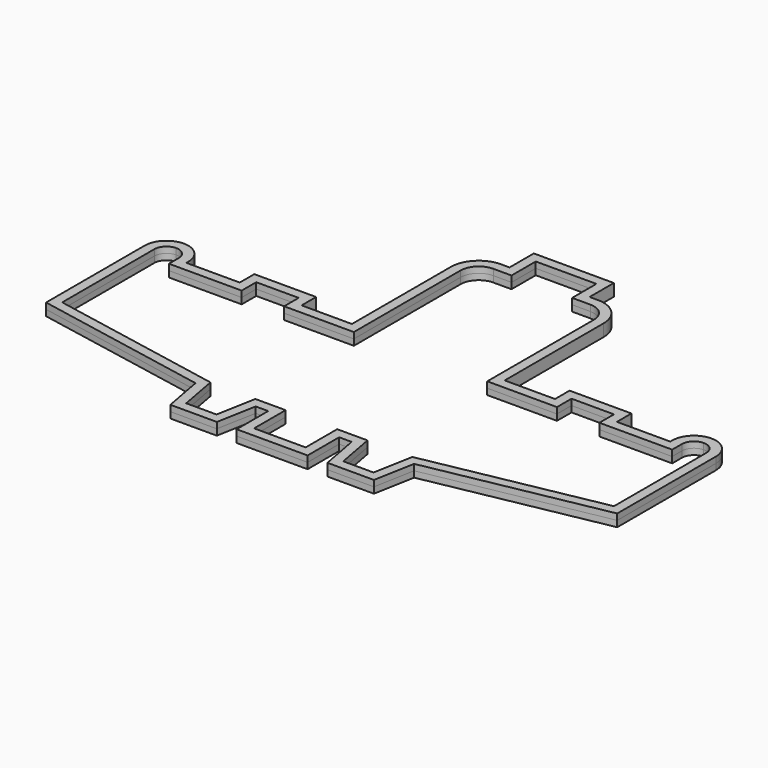
from build123d import *

# Parameters (mm, degrees)
F1_DEPTH = 1


# Not quite as in the source:
# - a feature names something its author has since deleted; it is built from what else it names


with BuildPart() as f1:
    # F0 (on Top) → F1 (new body, symmetric)
    with BuildSketch(Plane.XY):
        with BuildLine():
            Line((6.5999999642, 31.0999999642), (0, 31.0999999642))
            Line((0, 31.0999999642), (-6.5999999642, 31.0999999642))
            Line((-6.5999999642, 31.0999999642), (-6.5999999642, 26.0999999642))
            Line((-6.5999999642, 26.0999999642), (-8, 26.0999999642))
            ThreePointArc((-8, 26.0999999642), (-11.2526911682, 24.7526911682), (-12.5999999642, 21.5))
            Line((-12.5999999642, 21.5), (-12.5999999642, 1.0999999642))
            Line((-12.5999999642, 1.0999999642), (-20.9000000358, 1.0999999642))
            Line((-20.9000000358, 1.0999999642), (-20.9000000358, 4.0999999642))
            Line((-20.9000000358, 4.0999999642), (-31.0999999642, 4.0999999642))
            Line((-31.0999999642, 4.0999999642), (-31.0999999642, 1.0999999642))
            Line((-31.0999999642, 1.0999999642), (-39.922291276, 1.0999999642))
            ThreePointArc((-39.922291276, 1.0999999642), (-40.8167184403, 3.8999999613), (-43.5, 5.0999999642))
            ThreePointArc((-43.5, 5.0999999642), (-46.045584387, 4.045584387), (-47.0999999642, 1.5))
            Line((-47.0999999642, 1.5), (-47.0999999642, -18.823789758))
            Line((-47.0999999642, -18.823789758), (-18.0247169235, -24.366737998))
            Line((-18.0247169235, -24.366737998), (-16.7816531759, -31.0999999642))
            Line((-16.7816531759, -31.0999999642), (-9.1183468241, -31.0999999642))
            Line((-9.1183468241, -31.0999999642), (-7.9183468241, -24.5999999642))
            Line((-7.9183468241, -24.5999999642), (-5.8499999642, -24.5999999642))
            Line((-5.8499999642, -24.5999999642), (-5.8499999642, -31.0999999642))
            Line((-5.8499999642, -31.0999999642), (0, -31.0999999642))
            Line((0, -31.0999999642), (5.8499999642, -31.0999999642))
            Line((5.8499999642, -31.0999999642), (5.8499999642, -24.5999999642))
            Line((5.8499999642, -24.5999999642), (7.9183468241, -24.5999999642))
            Line((7.9183468241, -24.5999999642), (9.1183468241, -31.0999999642))
            Line((9.1183468241, -31.0999999642), (16.7816531759, -31.0999999642))
            Line((16.7816531759, -31.0999999642), (18.0247169235, -24.366737998))
            Line((18.0247169235, -24.366737998), (47.0999999642, -18.823789758))
            Line((47.0999999642, -18.823789758), (47.0999999642, 1.5))
            ThreePointArc((47.0999999642, 1.5), (46.045584387, 4.045584387), (43.5, 5.0999999642))
            ThreePointArc((43.5, 5.0999999642), (40.8167184403, 3.8999999613), (39.922291276, 1.0999999642))
            Line((39.922291276, 1.0999999642), (31.0999999642, 1.0999999642))
            Line((31.0999999642, 1.0999999642), (31.0999999642, 4.0999999642))
            Line((31.0999999642, 4.0999999642), (20.9000000358, 4.0999999642))
            Line((20.9000000358, 4.0999999642), (20.9000000358, 1.0999999642))
            Line((20.9000000358, 1.0999999642), (12.5999999642, 1.0999999642))
            Line((12.5999999642, 1.0999999642), (12.5999999642, 21.5))
            ThreePointArc((12.5999999642, 21.5), (11.2526911682, 24.7526911682), (8, 26.0999999642))
            Line((8, 26.0999999642), (6.5999999642, 26.0999999642))
            Line((6.5999999642, 26.0999999642), (6.5999999642, 31.0999999642))
        make_face()
        with BuildLine():
            Line((-5, 29.5), (0, 29.5))
            Line((0, 29.5), (5, 29.5))
            Line((5, 29.5), (5, 24.5))
            Line((5, 24.5), (8, 24.5))
            ThreePointArc((8, 24.5), (10.1213203436, 23.6213203436), (11, 21.5))
            Line((11, 21.5), (11, -0.5))
            Line((11, -0.5), (22.5, -0.5))
            Line((22.5, -0.5), (22.5, 2.5))
            Line((22.5, 2.5), (29.5, 2.5))
            Line((29.5, 2.5), (29.5, -0.5))
            Line((29.5, -0.5), (41.5, -0.5))
            Line((41.5, -0.5), (41.5, 1.5))
            ThreePointArc((41.5, 1.5), (42.0857864376, 2.9142135624), (43.5, 3.5))
            ThreePointArc((43.5, 3.5), (44.9142135624, 2.9142135624), (45.5, 1.5))
            Line((45.5, 1.5), (45.5, -17.5))
            Line((45.5, -17.5), (16.65, -23))
            Line((16.65, -23), (15.45, -29.5))
            Line((15.45, -29.5), (10.45, -29.5))
            Line((10.45, -29.5), (9.25, -23))
            Line((9.25, -23), (4.25, -23))
            Line((4.25, -23), (4.25, -29.5))
            Line((4.25, -29.5), (0, -29.5))
            Line((0, -29.5), (-4.25, -29.5))
            Line((-4.25, -29.5), (-4.25, -23))
            Line((-4.25, -23), (-9.25, -23))
            Line((-9.25, -23), (-10.45, -29.5))
            Line((-10.45, -29.5), (-15.45, -29.5))
            Line((-15.45, -29.5), (-16.65, -23))
            Line((-16.65, -23), (-45.5, -17.5))
            Line((-45.5, -17.5), (-45.5, 1.5))
            ThreePointArc((-45.5, 1.5), (-44.9142135624, 2.9142135624), (-43.5, 3.5))
            ThreePointArc((-43.5, 3.5), (-42.0857864376, 2.9142135624), (-41.5, 1.5))
            Line((-41.5, 1.5), (-41.5, -0.5))
            Line((-41.5, -0.5), (-29.5, -0.5))
            Line((-29.5, -0.5), (-29.5, 2.5))
            Line((-29.5, 2.5), (-22.5, 2.5))
            Line((-22.5, 2.5), (-22.5, -0.5))
            Line((-22.5, -0.5), (-11, -0.5))
            Line((-11, -0.5), (-11, 21.5))
            ThreePointArc((-11, 21.5), (-10.1213203436, 23.6213203436), (-8, 24.5))
            Line((-8, 24.5), (-5, 24.5))
            Line((-5, 24.5), (-5, 29.5))
        make_face(mode=Mode.SUBTRACT)
    extrude(amount=F1_DEPTH, both=True)


solid = f1.part
